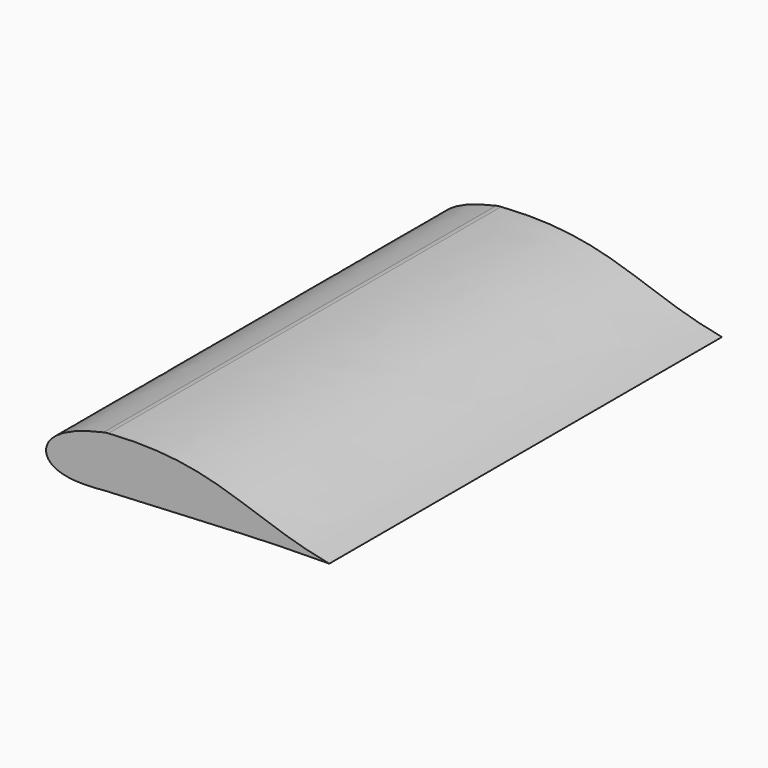
from build123d import *

# Parameters (mm, degrees)
F1_DEPTH = 70


# Not quite as in the source:
# - ends of sketch curves that miss each other by under 0.0002 mm in the source are joined


with BuildPart() as f1:
    # F0 (on Front) → F1 (new body)
    with BuildSketch(Plane.XZ):
        with BuildLine():
            ThreePointArc((8.4943538532, 6.1165723018), (8.1478009221, 6.0800981354), (7.80463009, 6.0195747612))
            add(Edge.make_bspline(
                [(7.80463009, 6.0195747612), (7.8033284675, 6.0192985857), (7.8020273177, 6.0190210249), (7.800726352, 6.018743432)],
                knots=[0.007555438, 0.007555438, 0.007555438, 0.007555438, 0.0076419863, 0.0076419863, 0.0076419863, 0.0076419863], degree=3))
            add(Edge.make_bspline(
                [(7.800726352, 6.018743432), (-0.0344115563, 4.3469248193), (-2.2359286822, -1.0520505926), (4.0699255085, -1.6493105494), (7.9768506791, -1.2445967448)],
                knots=[0.0076419863, 0.0076419863, 0.0076419863, 0.0076419863, 0.5288840216, 1, 1, 1, 1], degree=3))
            add(Edge.make_bspline(
                [(40, 0), (29.3975914618, 0), (19.3824759115, -0.7626691443), (7.9768506791, -1.2445967448)],
                knots=[0, 0, 0, 0, 32.0473261519, 32.0473261519, 32.0473261519, 32.0473261519], degree=3))
            add(Edge.make_bspline(
                [(8.4943538532, 6.1165723018), (23.7515253745, 7.1864547693), (28.0988142674, 2.2560978858), (40, 0)],
                knots=[0.2410904053, 0.2410904053, 0.2410904053, 0.2410904053, 32.4276209152, 32.4276209152, 32.4276209152, 32.4276209152], degree=3))
        make_face()
    extrude(amount=F1_DEPTH)


solid = f1.part
